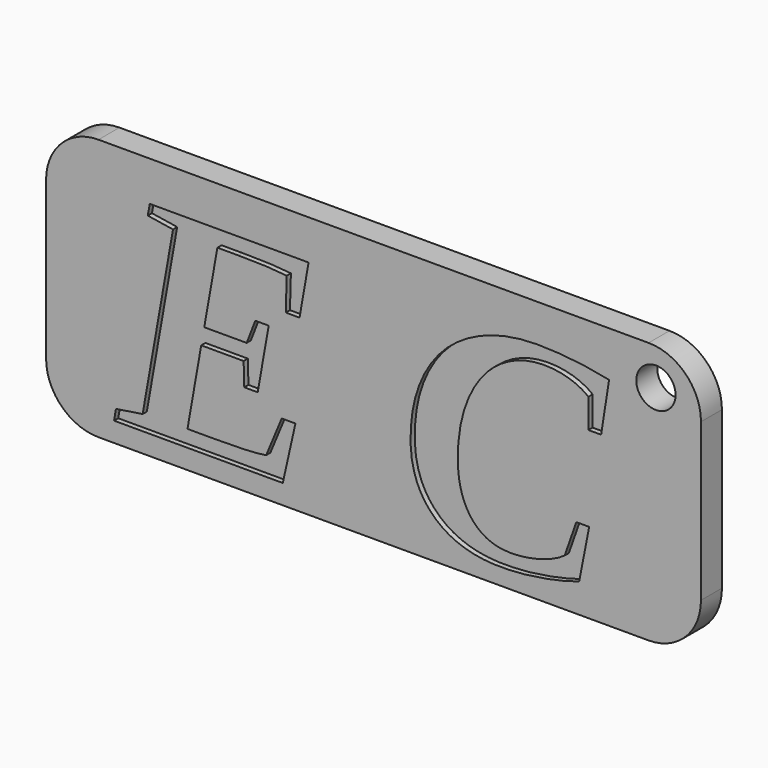
from build123d import *

# Parameters (mm, degrees)
F0_W         = 63.5
F0_H         = 25.4
F1_DEPTH     = 2.54
F2_TEXT_SIZE = 29.9861111111
F3_DEPTH     = 0.508
F4_R         = 5.08
F5_D         = 3.81
F5_DEPTH     = 12.7
F5_TIP       = 1.1446394792


# Not quite as in the source:
# - Text() gives the source's letters only with a copy of the font that has no kerning and outlines rounded to 1/6400 em; it was checked with that copy


with BuildPart() as f1:
    # F0 (on Front) → F1 (new body)
    with BuildSketch(Plane.XZ):
        Rectangle(F0_W, F0_H)
    extrude(amount=F1_DEPTH)

    # F2 (on face) → F3 (cut)
    with BuildSketch(Plane.XZ.offset(2.54)):
        with Locations((-24.9353255208, -10.795)):
            Text('E C', F2_TEXT_SIZE, font='Tinos', font_style=FontStyle.BOLDITALIC, text_align=(TextAlign.LEFT, TextAlign.BOTTOM))
    extrude(amount=-F3_DEPTH, mode=Mode.SUBTRACT)

    # F4
    f4_edges = [f1.edges().sort_by_distance(p)[0] for p in [
        (31.75, -1.27, 12.7),
        (31.75, -1.27, -12.7),
        (-31.75, -1.27, 12.7),
        (-31.75, -1.27, -12.7),
    ]]
    fillet(f4_edges, radius=F4_R)

    # F5
    with Locations(Plane(origin=(0, 0, 0), x_dir=(1, 0, 0), z_dir=(0, 1, 0))):
        with Locations((27.3840185255, -9.1046141461)):
            Hole(F5_D / 2, depth=F5_DEPTH)
            with Locations((0, 0, -(F5_DEPTH + F5_TIP / 2))):  # 118° drill point
                Cone(0, F5_D / 2, F5_TIP, mode=Mode.SUBTRACT)


solid = f1.part
